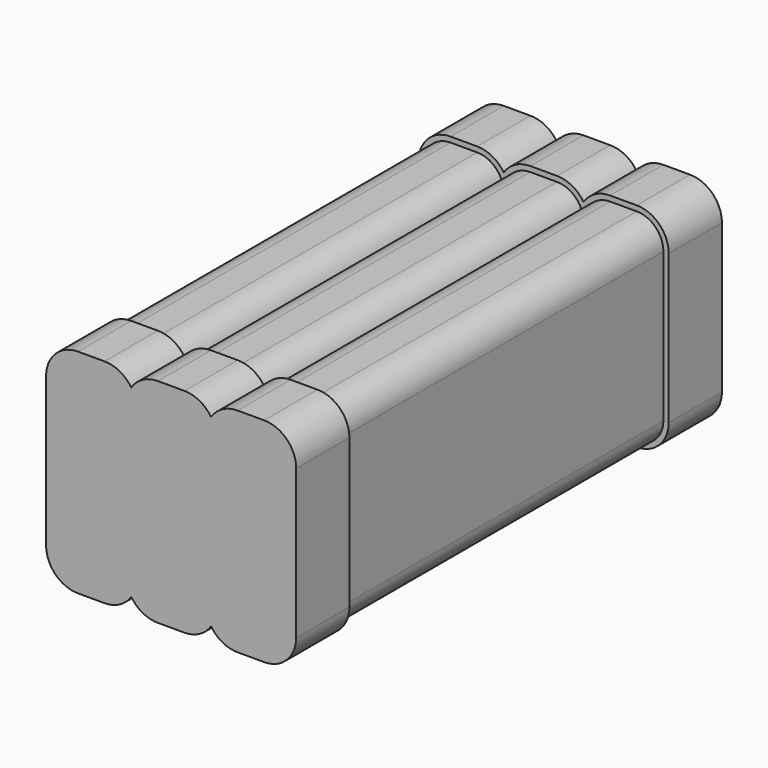
from build123d import *

# Parameters (mm, degrees)
F0_W     = 100
F0_H     = 76
F1_DEPTH = 30
F2_R     = 10
F5_W     = 115
F5_H     = 96
F5_W_2   = 100
F5_H_2   = 56
F6_DEPTH = 30
F8_DEPTH = 25


with BuildPart() as f1:
    # F0 (on Right) → F1 (new body)
    with BuildSketch(Plane.YZ):
        with Locations((50, 38)):
            Rectangle(F0_W, F0_H)
    extrude(amount=F1_DEPTH)

    # F2
    f2_edges = [f1.edges().sort_by_distance(p)[0] for p in [
        (30, 50, 76),
        (0, 50, 76),
        (30, 50, 0),
        (0, 50, 0),
    ]]
    fillet(f2_edges, radius=F2_R)

    # F3: F1 across face


with BuildPart() as f1_1:
    add(f1.part)
    add(f1.part.mirror(Plane(origin=(30, 50, 38), x_dir=(0, 1, 0), z_dir=(1, 0, 0))))

    # F4: F1 across face


with BuildPart() as f1_2:
    add(f1_1.part)
    add(f1_1.part.mirror(Plane(origin=(60, 50, 38), x_dir=(0, 1, 0), z_dir=(1, 0, 0))))

    # F5 (on face) → F6 (cut)
    with BuildSketch(Plane.YZ.offset(120)):
        with Locations((52.5, 38)):
            Rectangle(F5_W, F5_H)
        with Locations((50, 38)):
            Rectangle(F5_W_2, F5_H_2, mode=Mode.SUBTRACT)
        with Locations((50, 38)):
            Rectangle(F5_W_2, F5_H_2)
    extrude(amount=-F6_DEPTH, mode=Mode.SUBTRACT)

    # F7 (on face) → F8 (join)
    with BuildSketch(Plane.XZ):
        with BuildLine():
            ThreePointArc((60, 3.3667504193), (64.3254513381, -0.5735281474), (70, -2))
            Line((70, -2), (80, -2))
            ThreePointArc((80, -2), (88.4852813742, 1.5147186258), (92, 10))
            Line((92, 10), (92, 66))
            ThreePointArc((92, 66), (88.4852813742, 74.4852813742), (80, 78))
            Line((80, 78), (70, 78))
            ThreePointArc((70, 78), (64.3254513381, 76.5735281474), (60, 72.6332495807))
            ThreePointArc((60, 72.6332495807), (55.6745486619, 76.5735281474), (50, 78))
            Line((50, 78), (40, 78))
            ThreePointArc((40, 78), (34.3254513381, 76.5735281474), (30, 72.6332495807))
            ThreePointArc((30, 72.6332495807), (25.6745486619, 76.5735281474), (20, 78))
            Line((20, 78), (10, 78))
            ThreePointArc((10, 78), (1.5147186258, 74.4852813742), (-2, 66))
            Line((-2, 66), (-2, 10))
            ThreePointArc((-2, 10), (1.5147186258, 1.5147186258), (10, -2))
            Line((10, -2), (20, -2))
            ThreePointArc((20, -2), (25.6745486619, -0.5735281474), (30, 3.3667504193))
            ThreePointArc((30, 3.3667504193), (34.3254513381, -0.5735281474), (40, -2))
            Line((40, -2), (50, -2))
            ThreePointArc((50, -2), (55.6745486619, -0.5735281474), (60, 3.3667504193))
        make_face()
        with BuildLine():
            ThreePointArc((0, 66), (2.9289321881, 73.0710678119), (10, 76))
            Line((10, 76), (20, 76))
            ThreePointArc((20, 76), (27.0710678119, 73.0710678119), (30, 66))
            ThreePointArc((30, 66), (32.9289321881, 73.0710678119), (40, 76))
            Line((40, 76), (50, 76))
            ThreePointArc((50, 76), (57.0710678119, 73.0710678119), (60, 66))
            ThreePointArc((60, 66), (62.9289321881, 73.0710678119), (70, 76))
            Line((70, 76), (80, 76))
            ThreePointArc((80, 76), (87.0710678119, 73.0710678119), (90, 66))
            Line((90, 66), (90, 10))
            ThreePointArc((90, 10), (87.0710678119, 2.9289321881), (80, 0))
            Line((80, 0), (70, 0))
            ThreePointArc((70, 0), (62.9289321881, 2.9289321881), (60, 10))
            ThreePointArc((60, 10), (57.0710678119, 2.9289321881), (50, 0))
            Line((50, 0), (40, 0))
            ThreePointArc((40, 0), (32.9289321881, 2.9289321881), (30, 10))
            ThreePointArc((30, 10), (27.0710678119, 2.9289321881), (20, 0))
            Line((20, 0), (10, 0))
            ThreePointArc((10, 0), (2.9289321881, 2.9289321881), (0, 10))
            Line((0, 10), (0, 66))
        make_face(mode=Mode.SUBTRACT)
    extrude(amount=-F8_DEPTH)

    # F9: F1 across face


with BuildPart() as f1_3:
    add(f1_2.part)
    add(f1_2.part.mirror(Plane(origin=(45, 100, 38), x_dir=(-1, 0, 0), z_dir=(0, 1, 0))))


solid = f1_3.part
